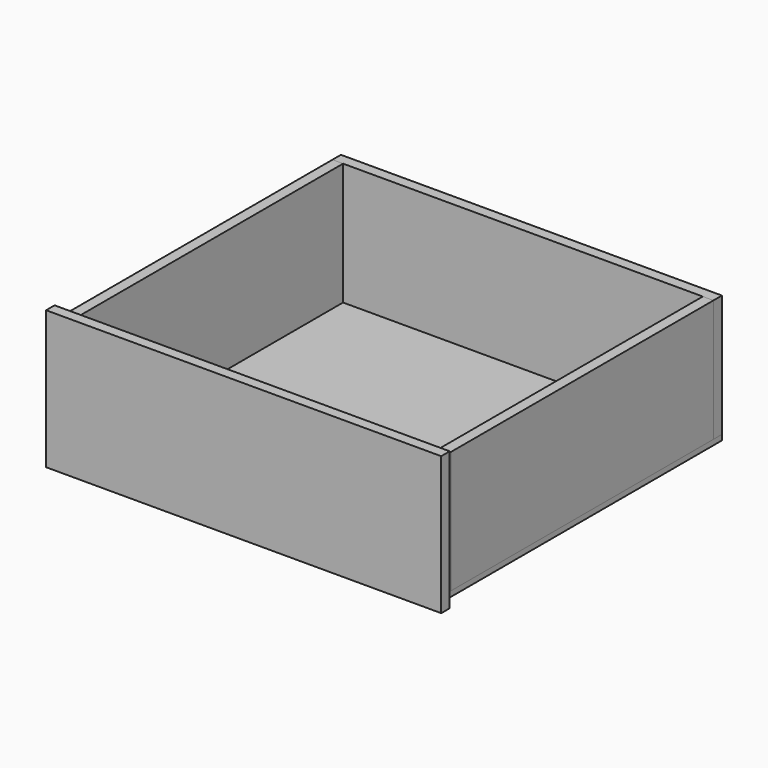
from build123d import *

# Parameters (mm, degrees)
F0_W     = 430
F0_H     = 138
F1_DEPTH = 12
F2_W     = 12
F2_H     = 138
F3_DEPTH = 370
F4_W     = 418
F4_H     = 138
F4_W_2   = 12
F5_DEPTH = 12
F6_W     = 12
F6_H     = 370
F7_DEPTH = 6
F8_W     = 446
F8_H     = 156
F8_W_2   = 430
F8_H_2   = 138
F9_DEPTH = 12


with BuildPart() as f1:
    # F0 (on Front) → F1 (new body)
    with BuildSketch(Plane.XZ):
        with Locations((210.308117494, 52.4257982135)):
            Rectangle(F0_W, F0_H)
    extrude(amount=F1_DEPTH)


with BuildPart() as f3:
    # F2 (on face) → F3 (new body)
    with BuildSketch(Plane.XZ.offset(12)):
        with Locations((1.308117494, 52.4257982135)):
            Rectangle(F2_W, F2_H)
    extrude(amount=F3_DEPTH)


with BuildPart() as f3b:
    # F2 (on face) → F3, piece 2 (new body)
    with BuildSketch(Plane.XZ.offset(12)):
        with Locations((419.308117494, 52.4257982135)):
            Rectangle(F2_W, F2_H)
    extrude(amount=F3_DEPTH)


with BuildPart() as f5:
    # F4 (on face) → F5 (new body)
    with BuildSketch(Plane.XZ.offset(382)):
        with Locations((216.308117494, 52.4257982135)):
            Rectangle(F4_W, F4_H)
        with Locations((1.308117494, 52.4257982135)):
            Rectangle(F4_W_2, F4_H)
    extrude(amount=F5_DEPTH)

    # F8 (on face) → F9 (join)
    with BuildSketch(Plane.XZ.offset(394)):
        with Locations((210.308117494, 51.4257982135)):
            Rectangle(F8_W, F8_H)
        with Locations((210.308117494, 52.4257982135)):
            Rectangle(F8_W_2, F8_H_2, mode=Mode.SUBTRACT)
        with Locations((210.308117494, 52.4257982135)):
            Rectangle(F8_W_2, F8_H_2)
    extrude(amount=F9_DEPTH)


with BuildPart() as f7:
    # F6 (on face) → F7 (new body)
    with BuildSketch(Plane(origin=(0, 0, -16.5742017865), x_dir=(1, 0, 0), z_dir=(0, 0, -1))):
        Polygon((425.308117494, 394), (-4.691882506, 394), (-4.691882506, 382), (7.308117494, 382), (7.308117494, 12), (425.308117494, 12), align=None)
        with Locations((1.308117494, 197)):
            Rectangle(F6_W, F6_H)
        Polygon((425.308117494, 0), (425.308117494, 12), (7.308117494, 12), (-4.691882506, 12), (-4.691882506, 0), align=None)
    extrude(amount=F7_DEPTH)


solid = Compound([f1.part, f3.part, f3b.part, f5.part, f7.part])
